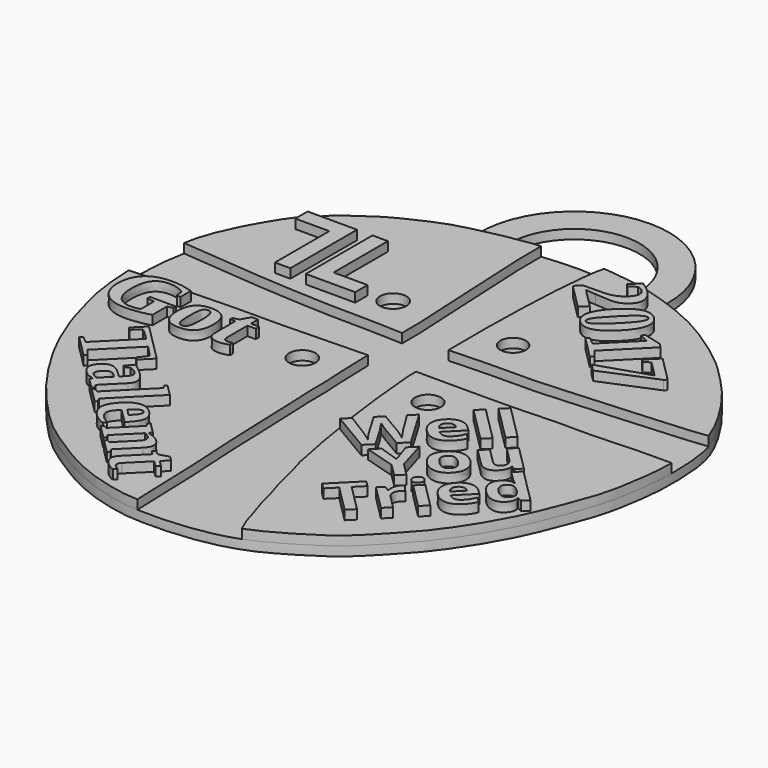
from build123d import *

# Parameters (mm, degrees)
F1_DEPTH     = 0.762
F2_R         = 1.0872392711
F2_R_2       = 1.0463116116
F2_R_3       = 1.0683652185
F2_R_4       = 1.0841442821
F3_DEPTH     = 0.762
F4_TEXT_SIZE = 7.0555555556
F5_TEXT_SIZE = 7.0555555556
F6_TEXT_SIZE = 5.2916666667
F8_DEPTH     = 0.762


# Not quite as in the source:
# - Text() gives the source's letters only with a copy of the font that has no kerning and outlines rounded to 1/6400 em; it was checked with that copy


with BuildPart() as f1:
    # F0 (on Top) → F1 (new body)
    with BuildSketch(Plane.XY):
        with BuildLine():
            add(Edge.make_bspline(
                [(2.6021334443, 18.9397180778), (2.3726177561, 18.961825666), (1.2318015764, 19.061867596), (-0.5497315274, 19.1653714447), (-2.4154644664, 19.0111404963), (-3.2044824224, 18.9380663852)],
                knots=[0.9593927449, 0.9593927449, 0.9593927449, 0.9593927449, 0.9638211084, 0.9818018096, 1, 1, 1, 1], degree=3))
            add(Edge.make_bspline(
                [(-3.2044824224, 18.9380663852), (-3.4183323449, 18.918260888), (-3.621203362, 18.8987863188), (-3.8163603922, 18.878384662)],
                knots=[0, 0, 0, 0, 0.0049323106, 0.0049323106, 0.0049323106, 0.0049323106], degree=3))
            Line((-3.8163603922, 18.878384662), (-5.9343413602, 18.5379368993))
            add(Edge.make_bspline(
                [(-5.9343413602, 18.5379368993), (-6.1595326867, 18.489820216), (-6.8628803931, 18.3355300315), (-7.7414437287, 18.1534983483), (-8.3188949184, 18.0136690301)],
                knots=[0.02400447, 0.02400447, 0.02400447, 0.02400447, 0.0298367152, 0.0413361445, 0.0413361445, 0.0413361445, 0.0413361445], degree=3))
            add(Edge.make_bspline(
                [(-8.3188949184, 18.0136690301), (-8.6991194979, 17.921597969), (-9.9490850785, 17.5896942369), (-11.5935376489, 16.8343890596), (-13.8352651313, 15.783666943), (-15.0452244767, 14.7583768617), (-16.2397073614, 14.1537516496), (-17.0754818626, 12.9719135809), (-18.0072673472, 12.3316469069), (-18.9744748049, 10.7820311318), (-20.0366911771, 8.9663186598), (-21.1032679215, 6.5193760274), (-21.3972730314, 4.8897056622), (-21.7892996847, 2.9127399495), (-21.8014501514, -0.2038543876), (-21.8021109531, -0.2259523709), (-21.7998947375, -0.252021435), (-21.7399832733, -2.0577578665), (-21.3670807921, -4.4871672329), (-20.8795181893, -6.0138065756), (-20.4674101598, -7.6732988429), (-19.7608032668, -9.4792625456), (-18.8007118231, -11.7388848932), (-16.5926192728, -15.3082276288), (-14.5758576004, -17.7452823316), (-12.3188829451, -20.1283447686), (-10.3173765434, -21.504691071), (-7.7727766541, -23.1180730298), (-5.4028423031, -24.0807446896), (-3.0685049826, -24.6432847968), (-1.4239719608, -24.8169850404), (2.2701085194, -24.7924292259), (6.3647743749, -23.9694522015), (9.287340819, -22.2974290413), (11.7110030318, -20.77747358), (13.089057831, -19.4578705132), (14.601932815, -17.858913696), (15.7505556728, -16.6061870854), (16.7620701924, -15.2117734965), (17.7759100984, -13.6957676313), (18.7530600709, -11.9707830872), (19.5257211385, -10.3932366067), (19.8938060185, -9.3727305593), (21.3032721983, -5.9698980302), (21.7794322385, -3.6154765788), (22.1118201442, -1.2754677713), (22.2180935616, 0.608131574), (22.1265496503, 2.8807821333), (21.8091160933, 5.1107971141), (20.3871562274, 7.8504658887), (18.6529194522, 10.3242858387), (16.9996684332, 12.001748683), (15.71935396, 13.3050522166), (13.7905470183, 14.7855683565), (11.0644407691, 16.5674424556), (8.7615671684, 17.4959878259), (7.4447259043, 17.9490330996), (7.1069626404, 18.057117434)],
                knots=[0.0413361445, 0.0413361445, 0.0413361445, 0.0413361445, 0.0489079805, 0.0663842972, 0.0839781053, 0.0981301872, 0.1110205303, 0.1243045862, 0.1362285738, 0.1511257584, 0.1679051855, 0.186213233, 0.2003875418, 0.217757122, 0.2367295542, 0.2376567093, 0.2386834765, 0.2528514088, 0.2715055772, 0.2857117794, 0.3002557717, 0.3157745727, 0.3335573714, 0.356590281, 0.3770868411, 0.3971780451, 0.4148785812, 0.4342995516, 0.4526104227, 0.4696961763, 0.4841583172, 0.5056153214, 0.5289248481, 0.5496955076, 0.5685289695, 0.5841617674, 0.6007577145, 0.6155412665, 0.6302062643, 0.6454768604, 0.6615894293, 0.6761413673, 0.6880987724, 0.7094189792, 0.7275698191, 0.7445541998, 0.7601242489, 0.7769449248, 0.7938505779, 0.8135968595, 0.8334146162, 0.8505661667, 0.8656331933, 0.883109424, 0.9035413595, 0.9236512547, 0.9305042241, 0.9305042241, 0.9305042241, 0.9305042241], degree=3))
            add(Edge.make_bspline(
                [(7.1069626404, 18.057117434), (6.4635369499, 18.2630138263), (5.6831685862, 18.477923721), (4.8610699056, 18.6347382733), (4.7278374742, 18.658628251)],
                knots=[0.9305042241, 0.9305042241, 0.9305042241, 0.9305042241, 0.9435588603, 0.9460677971, 0.9460677971, 0.9460677971, 0.9460677971], degree=3))
            Line((4.7278374742, 18.658628251), (2.6021334443, 18.9397180778))
        make_face()
        with BuildLine():
            add(Edge.make_bspline(
                [(-5.9343413602, 18.5379368993), (-6.1595326867, 18.489820216), (-6.8628803931, 18.3355300315), (-7.7414437287, 18.1534983483), (-8.3188949184, 18.0136690301)],
                knots=[0.02400447, 0.02400447, 0.02400447, 0.02400447, 0.0298367152, 0.0413361445, 0.0413361445, 0.0413361445, 0.0413361445], degree=3))
            ThreePointArc((-5.9343413602, 18.5379368993), (-0.6695923404, 24.4589608358), (4.7278374742, 18.658628251))
            add(Edge.make_bspline(
                [(7.1069626404, 18.057117434), (6.4635369499, 18.2630138263), (5.6831685862, 18.477923721), (4.8610699056, 18.6347382733), (4.7278374742, 18.658628251)],
                knots=[0.9305042241, 0.9305042241, 0.9305042241, 0.9305042241, 0.9435588603, 0.9460677971, 0.9460677971, 0.9460677971, 0.9460677971], degree=3))
            ThreePointArc((7.1069626404, 18.057117434), (-0.6309075054, 26.8905393576), (-8.3188949184, 18.0136690301))
        make_face()
    extrude(amount=F1_DEPTH)

    # F2 (on face) → F3 (join)
    with BuildSketch(Plane.XY.offset(0.762)):
        with BuildLine():
            add(Edge.make_bspline(
                [(-3.2044824224, 18.9380663852), (-3.2151950929, 18.257697419), (-3.2352822899, 16.9819459204), (-3.1018820595, 15.4611967516), (-3.0488706717, 14.1189178674), (-3.0051146695, 12.6676148971), (-2.9139271075, 11.0046560801), (-2.8329012419, 9.2443978743), (-2.7600732056, 7.5626014392), (-2.623822916, 5.6559492355), (-2.6328673275, 4.4915199718), (-2.6372846227, 3.9228121224)],
                knots=[0, 0, 0, 0, 0.1211948243, 0.2272509276, 0.3262920226, 0.4297486322, 0.5412587705, 0.6554826828, 0.7676773762, 0.8865335115, 1, 1, 1, 1], degree=3))
            add(Edge.make_bspline(
                [(-3.2044824224, 18.9380663852), (-3.4183323449, 18.918260888), (-3.621203362, 18.8987863188), (-3.8163603922, 18.878384662)],
                knots=[0, 0, 0, 0, 0.0049323106, 0.0049323106, 0.0049323106, 0.0049323106], degree=3))
            Line((-3.8163603922, 18.878384662), (-5.9343413602, 18.5379368993))
            add(Edge.make_bspline(
                [(-5.9343413602, 18.5379368993), (-6.1595326867, 18.489820216), (-6.8628803931, 18.3355300315), (-7.7414437287, 18.1534983483), (-8.3188949184, 18.0136690301)],
                knots=[0.02400447, 0.02400447, 0.02400447, 0.02400447, 0.0298367152, 0.0413361445, 0.0413361445, 0.0413361445, 0.0413361445], degree=3))
            add(Edge.make_bspline(
                [(-8.3188949184, 18.0136690301), (-8.6991194979, 17.921597969), (-9.9490850785, 17.5896942369), (-11.5935376489, 16.8343890596), (-13.8352651313, 15.783666943), (-15.0452244767, 14.7583768617), (-16.2397073614, 14.1537516496), (-17.0754818626, 12.9719135809), (-18.0072673472, 12.3316469069), (-18.9744748049, 10.7820311318), (-20.0366911771, 8.9663186598), (-21.1032679215, 6.5193760274), (-21.2948347774, 5.4575209184), (-21.3902935397, 4.9531100723)],
                knots=[0.0413361445, 0.0413361445, 0.0413361445, 0.0413361445, 0.0489079805, 0.0663842972, 0.0839781053, 0.0981301872, 0.1110205303, 0.1243045862, 0.1362285738, 0.1511257584, 0.1679051855, 0.186213233, 0.2003875418, 0.2003875418, 0.2003875418, 0.2003875418], degree=3))
            add(Edge.make_bspline(
                [(-21.3902935397, 4.9531100723), (-20.2709955922, 4.8740273818), (-17.9308101941, 4.6538628197), (-14.1240776513, 4.3145996398), (-11.6881931174, 4.1917231177), (-9.2241200689, 4.0374575392), (-6.397112284, 4.059071965), (-4.4246536732, 3.9800419874), (-3.2193934059, 3.9414454989), (-2.6372846227, 3.9228121224)],
                knots=[0, 0, 0, 0, 0.164799448, 0.3365124468, 0.4735972427, 0.6114586014, 0.7595242658, 0.8835195636, 1, 1, 1, 1], degree=3))
        make_face()
        with Locations((-5.8506716054, 7.0251724157)):
            Circle(F2_R, mode=Mode.SUBTRACT)
        with BuildLine():
            add(Edge.make_bspline(
                [(2.6021334443, 18.9397180778), (2.3726177561, 18.961825666), (2.1471755622, 18.9815954349), (1.927891, 18.9996889732)],
                knots=[0.9593927449, 0.9593927449, 0.9593927449, 0.9593927449, 0.9638211084, 0.9638211084, 0.9638211084, 0.9638211084], degree=3))
            add(Edge.make_bspline(
                [(1.927891, 18.9996889732), (1.8807769046, 18.8283249862), (1.7631076465, 18.4003368633), (1.5956989437, 17.0306026337), (1.5324690135, 15.9690695899), (1.3709819372, 14.6077769779), (1.3506777064, 13.2915061295), (1.2195471247, 11.6203655517), (1.2545442508, 9.8591836455), (1.1501829418, 8.2511163895), (1.1806183534, 6.7481668045), (1.1705269619, 5.2456414046), (1.17731392, 4.3541548115), (1.1805977662, 3.9228121224)],
                knots=[0, 0, 0, 0, 0.0607187049, 0.1516472917, 0.2343178806, 0.3243593956, 0.4145045793, 0.5154772297, 0.6197581496, 0.7188379355, 0.8146820052, 0.9103345324, 1, 1, 1, 1], degree=3))
            add(Edge.make_bspline(
                [(1.1805977662, 3.9228121224), (1.779962259, 3.9519939558), (2.8886301061, 4.005972387), (4.2118732129, 4.041096464), (5.4576221627, 4.0198694758), (7.8884345493, 4.0404425531), (9.7966192937, 4.1440386714), (11.1880965857, 4.2579476948), (12.970060195, 4.3770375545), (14.8442083134, 4.4985045839), (16.4324099803, 4.591781192), (18.1252516298, 4.7529786306), (20.0833963789, 4.8415795456), (21.5049901968, 5.0073097442), (21.6270957131, 5.0392108443), (21.6759156425, 5.0454488429)],
                knots=[0, 0, 0, 0, 0.0826460002, 0.1534869659, 0.2234521246, 0.3214124987, 0.4088764827, 0.4822429384, 0.5658192821, 0.6522031862, 0.7309614081, 0.8124456357, 0.9035072253, 0.9755516368, 1, 1, 1, 1], degree=3))
            add(Edge.make_bspline(
                [(21.6759156425, 5.0454488429), (21.3834158703, 5.9309873574), (20.3871562274, 7.8504658887), (18.6529194522, 10.3242858387), (16.9996684332, 12.001748683), (15.71935396, 13.3050522166), (13.7905470183, 14.7855683565), (11.0644407691, 16.5674424556), (8.7615671684, 17.4959878259), (7.4447259043, 17.9490330996), (7.1069626404, 18.057117434)],
                knots=[0.7938505779, 0.7938505779, 0.7938505779, 0.7938505779, 0.8135968595, 0.8334146162, 0.8505661667, 0.8656331933, 0.883109424, 0.9035413595, 0.9236512547, 0.9305042241, 0.9305042241, 0.9305042241, 0.9305042241], degree=3))
            add(Edge.make_bspline(
                [(7.1069626404, 18.057117434), (6.4635369499, 18.2630138263), (5.6831685862, 18.477923721), (4.8610699056, 18.6347382733), (4.7278374742, 18.658628251)],
                knots=[0.9305042241, 0.9305042241, 0.9305042241, 0.9305042241, 0.9435588603, 0.9460677971, 0.9460677971, 0.9460677971, 0.9460677971], degree=3))
            Line((4.7278374742, 18.658628251), (2.6021334443, 18.9397180778))
        make_face()
        with Locations((4.0059808631, 7.0355138215)):
            Circle(F2_R_2, mode=Mode.SUBTRACT)
        with BuildLine():
            add(Edge.make_bspline(
                [(6.3258755941, -23.7647709963), (7.4475861777, -23.3499670856), (9.287340819, -22.2974290413), (11.7110030318, -20.77747358), (13.089057831, -19.4578705132), (14.601932815, -17.858913696), (15.7505556728, -16.6061870854), (16.7620701924, -15.2117734965), (17.7759100984, -13.6957676313), (18.7530600709, -11.9707830872), (19.5257211385, -10.3932366067), (19.8938060185, -9.3727305593), (21.3032721983, -5.9698980302), (21.7794322385, -3.6154765788), (22.1118201442, -1.2754677713), (22.1818892703, -0.0335564512), (22.1853937943, 0.6199455294)],
                knots=[0.5289248481, 0.5289248481, 0.5289248481, 0.5289248481, 0.5496955076, 0.5685289695, 0.5841617674, 0.6007577145, 0.6155412665, 0.6302062643, 0.6454768604, 0.6615894293, 0.6761413673, 0.6880987724, 0.7094189792, 0.7275698191, 0.7445541998, 0.7601242489, 0.7601242489, 0.7601242489, 0.7601242489], degree=3))
            add(Edge.make_bspline(
                [(22.1853937943, 0.6199455294), (21.5901705458, 0.6280927016), (20.2925124467, 0.6458547993), (17.6460766265, 0.5044090269), (15.9450809618, 0.4251590495), (14.3214294026, 0.4065279667), (12.4829632776, 0.4671208319), (10.4949012445, 0.3279817639), (8.7854144561, 0.2870905739), (6.6454745613, 0.3151066799), (5.1734368889, 0.2538998733), (3.5952954099, 0.2889488476), (2.4633578723, 0.2841900844), (1.7626285699, 0.2819964835), (1.4231849451, 0.2843155)],
                knots=[0, 0, 0, 0, 0.0879432053, 0.1917472106, 0.2755602348, 0.3557089957, 0.4426219486, 0.5322570998, 0.6167526886, 0.7092985773, 0.7879546552, 0.867321643, 0.935475537, 1, 1, 1, 1], degree=3))
            add(Edge.make_bspline(
                [(1.4231849451, 0.2843155), (1.4178863232, 0.083814538), (1.4062405007, -0.356865062), (1.5033701488, -1.2716519815), (1.5649034335, -2.0047979454), (1.6526770754, -2.8869479744), (1.7484273783, -4.0489120184), (2.0214552259, -5.8542770167), (2.1661012607, -7.4029961043), (2.4818541911, -8.8193365643), (2.691049014, -10.1659805075), (2.8500610593, -11.1900287145), (3.1100664291, -12.3827397195), (3.3284234119, -13.3912412643), (3.3955476924, -14.0678474018), (3.5040687759, -14.3777137217)],
                knots=[0, 0, 0, 0, 0.0581030661, 0.1276148826, 0.1904863847, 0.2576394847, 0.3365820923, 0.4351415164, 0.5267573656, 0.6144065825, 0.6988117035, 0.7732500257, 0.8531287183, 0.9275777787, 1, 1, 1, 1], degree=3))
            add(Edge.make_bspline(
                [(3.5040687759, -14.3777137217), (3.6066118398, -14.7101977045), (3.8135186169, -15.3810689142), (4.0260002618, -16.4146467888), (4.4007872187, -17.8504825765), (4.7941517838, -18.9215462711), (4.9885300303, -20.0426897698), (5.396118977, -20.994701844), (5.6672346742, -22.045691971), (5.8906796926, -22.8303723607), (6.1754392457, -23.4417727369), (6.3258755941, -23.7647709963)],
                knots=[0, 0, 0, 0, 0.1084531231, 0.2188318285, 0.3484026693, 0.4635516475, 0.5758634478, 0.6851576, 0.7953468741, 0.8918832797, 1, 1, 1, 1], degree=3))
        make_face()
        with Locations((4.6878579993, -2.5661294875)):
            Circle(F2_R_3, mode=Mode.SUBTRACT)
        with BuildLine():
            add(Edge.make_bspline(
                [(-21.8015879403, -0.2343613249), (-21.4530127708, -0.2076276136), (-20.7062698129, -0.1503562871), (-19.3387956765, -0.1846235709), (-17.2463907929, -0.1846187329), (-15.1463944702, -0.0928971289), (-11.7497558491, -0.0206729644), (-9.738864802, -0.0676512435), (-7.1178899846, 0.0590452552), (-4.9685458918, 0.0758000823), (-3.2606691441, 0.129328912), (-2.4257365625, 0.1416163924)],
                knots=[0, 0, 0, 0, 0.0791831449, 0.1688107468, 0.2781703597, 0.3920089754, 0.5316904784, 0.6428606796, 0.7646119079, 0.8783755491, 1, 1, 1, 1], degree=3))
            add(Edge.make_bspline(
                [(-21.8015879403, -0.2343613249), (-21.7980773908, -0.3067964126), (-21.7399832733, -2.0577578665), (-21.3670807921, -4.4871672329), (-20.8795181893, -6.0138065756), (-20.4674101598, -7.6732988429), (-19.7608032668, -9.4792625456), (-18.8007118231, -11.7388848932), (-16.5926192728, -15.3082276288), (-14.5758576004, -17.7452823316), (-12.3188829451, -20.1283447686), (-10.3173765434, -21.504691071), (-7.7727766541, -23.1180730298), (-5.4028423031, -24.0807446896), (-3.0685049826, -24.6432847968), (-2.0896982009, -24.7466691461), (-1.458483563, -24.7725663301)],
                knots=[0.2386834765, 0.2386834765, 0.2386834765, 0.2386834765, 0.2528514088, 0.2715055772, 0.2857117794, 0.3002557717, 0.3157745727, 0.3335573714, 0.356590281, 0.3770868411, 0.3971780451, 0.4148785812, 0.4342995516, 0.4526104227, 0.4696961763, 0.4841583172, 0.4841583172, 0.4841583172, 0.4841583172], degree=3))
            add(Edge.make_bspline(
                [(-2.4257365625, 0.1416163924), (-2.4005302952, -0.276031696), (-2.3495304026, -1.1210599347), (-2.3640704517, -2.4428693112), (-2.2792035945, -3.7863967616), (-2.1971856671, -5.0733635503), (-2.2487168296, -6.0552120179), (-2.1671378005, -7.2813681108), (-2.1289923847, -8.3615045414), (-2.0497123297, -11.0618449424), (-1.9405508812, -13.5550937082), (-1.8739997833, -15.1528311227), (-1.7450303592, -17.8520320714), (-1.6458173916, -18.9710557417), (-1.5826946846, -20.6526126326), (-1.5813719174, -21.6728622351), (-1.4982206972, -23.1200005656), (-1.472122753, -24.205347306), (-1.458483563, -24.7725663301)],
                knots=[0, 0, 0, 0, 0.0569761046, 0.11527987, 0.1745706627, 0.2317833015, 0.2824956045, 0.3372634386, 0.3903656045, 0.4737485539, 0.5542096763, 0.6200051788, 0.7017753922, 0.7578574051, 0.8218765824, 0.8739631858, 0.9341312079, 1, 1, 1, 1], degree=3))
        make_face()
        with Locations((-5.4736498754, -2.7894569156)):
            Circle(F2_R_4, mode=Mode.SUBTRACT)
    extrude(amount=F3_DEPTH)

    # F4 (on face) + F5 (on face) + F6 (on face) + F7 (on face) → F8 (join)
    with BuildSketch(Plane.XY.offset(1.524)):
        with Locations(Location((2.5358654148, 14.958166722), (0, 0, -45))):
            Text('2017', F4_TEXT_SIZE, font='Tinos', font_style=FontStyle.BOLD, text_align=(TextAlign.LEFT, TextAlign.BOTTOM))
    with BuildSketch(Plane.XY.offset(1.524)):
        with Locations((-20.6650607639, -5.5052848881)):
            Text('Got', F5_TEXT_SIZE, font='Tinos', font_style=FontStyle.BOLD, text_align=(TextAlign.LEFT, TextAlign.BOTTOM))
        with Locations(Location((-18.3241024484, -9.8593873365), (0, 0, -45))):
            Text('Talent', F5_TEXT_SIZE, font='Tinos', font_style=FontStyle.BOLD, text_align=(TextAlign.LEFT, TextAlign.BOTTOM))
    with BuildSketch(Plane.XY.offset(1.524)):
        with Locations(Location((5.2821356592, -11.6884355755), (0, 0, 45))):
            Text('Well', F6_TEXT_SIZE, font='Open Sans', font_style=FontStyle.BOLD, text_align=(TextAlign.LEFT, TextAlign.BOTTOM))
        with Locations(Location((9.3595862628, -13.8833783849), (0, 0, 45))):
            Text('You', F6_TEXT_SIZE, font='Open Sans', font_style=FontStyle.BOLD, text_align=(TextAlign.LEFT, TextAlign.BOTTOM))
        with Locations(Location((9.9600849615, -19.5332874277), (0, 0, 45))):
            Text('Tried', F6_TEXT_SIZE, font='Open Sans', font_style=FontStyle.BOLD, text_align=(TextAlign.LEFT, TextAlign.BOTTOM))
    with BuildSketch(Plane.XY.offset(1.524)):
        Polygon((-10.414, 12.192), (-11.684, 12.192), (-11.684, 5.334), (-7.62, 5.334), (-7.62, 6.604), (-10.414, 6.604), align=None)
        Polygon((-12.954, 5.334), (-12.954, 12.192), (-17.018, 12.192), (-17.018, 10.922), (-14.224, 10.922), (-14.224, 5.334), align=None)
    extrude(amount=F8_DEPTH)


solid = f1.part
